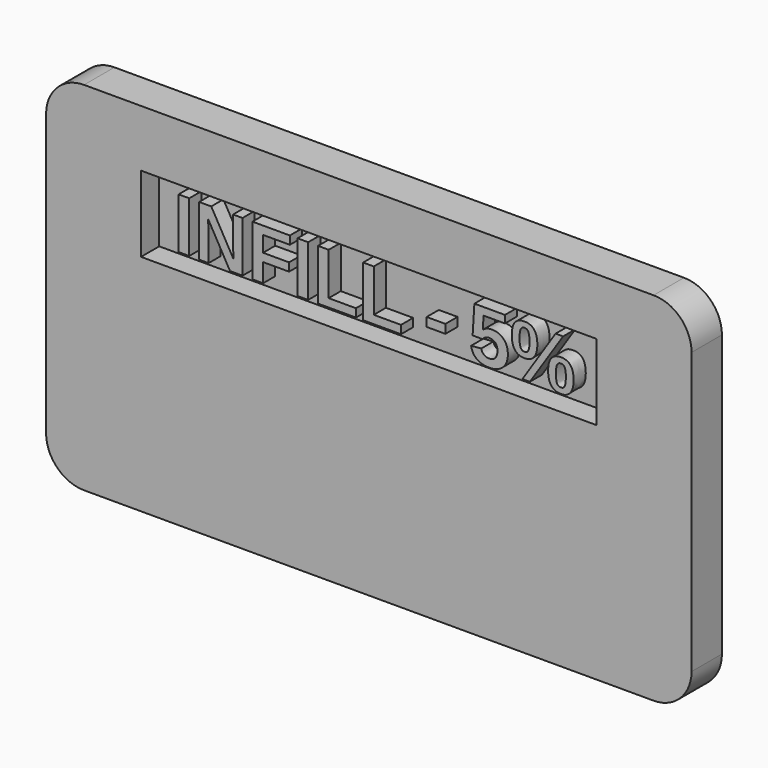
from build123d import *

# Parameters (mm, degrees)
F0_W         = 85
F0_H         = 47
F0_W_2       = 60
F0_H_2       = 10
F1_DEPTH     = 5
F2_DEPTH     = 2
F3_TEXT_SIZE = 9.7222222222
F4_DEPTH     = 2
F5_R         = 5


# Not quite as in the source:
# - Text() gives the source's letters only with a copy of the font that has no kerning and outlines rounded to 1/6400 em; it was checked with that copy


with BuildPart() as f1:
    # F0 (on Front) → F1 (new body)
    with BuildSketch(Plane.XZ):
        Rectangle(F0_W, F0_H)
        with Locations((0, 11)):
            Rectangle(F0_W_2, F0_H_2, mode=Mode.SUBTRACT)
    extrude(amount=F1_DEPTH)

    # F0 (on Front) → F2 (join)
    with BuildSketch(Plane.XZ):
        with Locations((0, 11)):
            Rectangle(F0_W_2, F0_H_2)
    extrude(amount=F2_DEPTH)

    # F3 (on face) → F4 (join)
    with BuildSketch(Plane.XZ.offset(2)):
        with Locations((-26.5, 7.5)):
            Text('INFILL - 5%', F3_TEXT_SIZE, font='Arimo', font_style=FontStyle.BOLD, text_align=(TextAlign.LEFT, TextAlign.BOTTOM))
    extrude(amount=F4_DEPTH)

    # F5
    f5_edges = [f1.edges().sort_by_distance(p)[0] for p in [
        (-42.5, -2.5, 23.5),
        (-42.5, -2.5, -23.5),
        (42.5, -2.5, 23.5),
        (42.5, -2.5, -23.5),
    ]]
    fillet(f5_edges, radius=F5_R)


solid = f1.part
